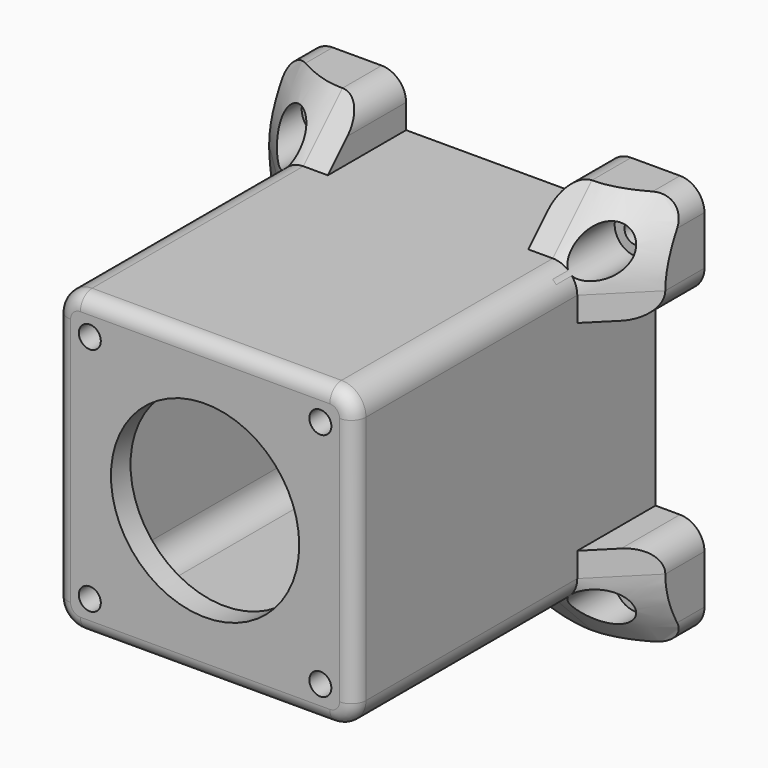
from build123d import *

# Parameters (mm, degrees)
F0_W          = 58
F0_H          = 58
F3_DEPTH      = 77
F4_DEPTH      = 5
F5_START      = 72
F0_R          = 19.25
F5_DEPTH      = 5
F6_DEPTH      = 91.6
F7_R          = 5
F8_D          = 4.5
F9_R          = 3
F10_T4_ANGLE  = 90
F10_T10_ANGLE = 90
F10_T16_ANGLE = 90
F10_T22_ANGLE = 90
F10_T28_DEPTH = 5
F10_T33_DEPTH = 5
F10_T38_DEPTH = 5
F10_T43_DEPTH = 5
F10_T48_DEPTH = 5
F10_T53_DEPTH = 5
F10_T58_DEPTH = 5
F10_T63_DEPTH = 5
F11_D         = 4.5
F13_START     = 7
F12_R         = 4.25
F13_DEPTH     = 17
F14_R         = 5


# Not quite as in the source:
# - a fillet or chamfer that OpenCascade refuses, or shapes differently, is made with other operations: its cross-section is extruded or revolved along the edge and cut away or added


with BuildPart() as f3:
    # F0 (on Front) → F3 (new body)
    with BuildSketch(Plane.XZ):
        Polygon((-30.5, -20.5), (-30.5, -30.5), (-20.5, -30.5), (20.5, -30.5), (30.5, -30.5), (30.5, -20.5), (30.5, 20.5), (30.5, 30.5), (20.5, 30.5), (-20.5, 30.5), (-30.5, 30.5), (-30.5, 20.5), align=None)
        Rectangle(F0_W, F0_H, mode=Mode.SUBTRACT)
    extrude(amount=F3_DEPTH)

    # F0 (on Front) → F4 (join)
    with BuildSketch(Plane.XZ):
        Polygon((-40.5, 20.5), (-30.5, 20.5), (-30.5, 30.5), (-20.5, 30.5), (-20.5, 40.5), (-40.5, 40.5), align=None)
        Polygon((30.5, 30.5), (30.5, 20.5), (40.5, 20.5), (40.5, 40.5), (20.5, 40.5), (20.5, 30.5), align=None)
        Polygon((30.5, -30.5), (20.5, -30.5), (20.5, -40.5), (40.5, -40.5), (40.5, -20.5), (30.5, -20.5), align=None)
        Polygon((-20.5, -30.5), (-30.5, -30.5), (-30.5, -20.5), (-40.5, -20.5), (-40.5, -40.5), (-20.5, -40.5), align=None)
    extrude(amount=F4_DEPTH)

    # F0 (on Front) → F5 (join)
    with BuildSketch(Plane.XZ.offset(F5_START)):
        Polygon((-30.5, -20.5), (-30.5, -30.5), (-20.5, -30.5), (20.5, -30.5), (30.5, -30.5), (30.5, -20.5), (30.5, 20.5), (30.5, 30.5), (20.5, 30.5), (-20.5, 30.5), (-30.5, 30.5), (-30.5, 20.5), align=None)
        Rectangle(F0_W, F0_H, mode=Mode.SUBTRACT)
        Rectangle(F0_W, F0_H)
        Circle(F0_R, mode=Mode.SUBTRACT)
    extrude(amount=F5_DEPTH)

    # F0 (on Front) → F6 (cut)
    with BuildSketch(Plane.XZ):
        Circle(F0_R)
    extrude(amount=F6_DEPTH, mode=Mode.SUBTRACT)

    # F7
    f7_edges = [f3.edges().sort_by_distance(p)[0] for p in [
        (-30.5, -41, 30.5),
        (-30.5, -41, -30.5),
        (30.5, -41, -30.5),
        (30.5, -41, 30.5),
        (-29, -36, -29),
        (-29, -36, 29),
        (29, -36, 29),
        (29, -36, -29),
    ]]
    fillet(f7_edges, radius=F7_R)

    # F8 (through all)
    with Locations(Plane(origin=(0, 0, 0), x_dir=(1, 0, 0), z_dir=(0, 1, 0))):
        with Locations((23.57, -23.57), (-23.57, 23.57), (-23.57, -23.57), (23.57, 23.57)):
            Hole(F8_D / 2)

    # F9
    f9_edges = [f3.edges().sort_by_distance(p)[0] for p in [
        (-30.5, -77, 0),
    ]]
    fillet(f9_edges, radius=F9_R)

    # F10: chamfer of 15 on 4 edges, made by hand


with BuildPart() as f10_tool2:
    # F10_s3 → F10_t4 (revolve)
    with BuildSketch(Plane.XY.offset(-25.5)):
        Polygon((30.5, -20), (45.5, -5), (30.5, -5), align=None)
    revolve(axis=Axis((25.5, -5, -25.5), (0, 1, 0)), revolution_arc=F10_T4_ANGLE)

    split(bisect_by=Plane.XY.offset(-40.5), keep=Keep.TOP)

    split(bisect_by=Plane.YZ.offset(40.5), keep=Keep.BOTTOM)


with BuildPart() as f3_1:
    add(f3.part)

    # F10_t1: union F10_tool2
    add(f10_tool2.part)


with BuildPart() as f10_tool8:
    # F10_s9 → F10_t10 (revolve)
    with BuildSketch(Plane.XY.offset(25.5)):
        Polygon((30.5, -20), (45.5, -5), (30.5, -5), align=None)
    revolve(axis=Axis((25.5, -5, 25.5), (0, -1, 0)), revolution_arc=F10_T10_ANGLE)

    split(bisect_by=Plane.YZ.offset(40.5), keep=Keep.BOTTOM)

    split(bisect_by=Plane.XY.offset(40.5), keep=Keep.BOTTOM)


with BuildPart() as f3_2:
    add(f3_1.part)

    # F10_t7: union F10_tool8
    add(f10_tool8.part)


with BuildPart() as f10_tool14:
    # F10_s15 → F10_t16 (revolve)
    with BuildSketch(Plane.XY.offset(25.5)):
        Polygon((-30.5, -20), (-45.5, -5), (-30.5, -5), align=None)
    revolve(axis=Axis((-25.5, -5, 25.5), (0, 1, 0)), revolution_arc=F10_T16_ANGLE)

    split(bisect_by=Plane.YZ.offset(-40.5), keep=Keep.TOP)

    split(bisect_by=Plane.XY.offset(40.5), keep=Keep.BOTTOM)


with BuildPart() as f3_3:
    add(f3_2.part)

    # F10_t13: union F10_tool14
    add(f10_tool14.part)


with BuildPart() as f10_tool20:
    # F10_s21 → F10_t22 (revolve)
    with BuildSketch(Plane.XY.offset(-25.5)):
        Polygon((-30.5, -20), (-45.5, -5), (-30.5, -5), align=None)
    revolve(axis=Axis((-25.5, -5, -25.5), (0, -1, 0)), revolution_arc=F10_T22_ANGLE)

    split(bisect_by=Plane.XY.offset(-40.5), keep=Keep.TOP)

    split(bisect_by=Plane.YZ.offset(-40.5), keep=Keep.TOP)


with BuildPart() as f3_4:
    add(f3_3.part)

    # F10_t19: union F10_tool20
    add(f10_tool20.part)


with BuildPart() as f10_tool26:
    # F10_s27 → F10_t28 (new body)
    with BuildSketch(Plane.XY.offset(-25.5)):
        Polygon((-30.5, -20), (-45.5, -5), (-30.5, -5), align=None)
    extrude(amount=F10_T28_DEPTH)

    split(bisect_by=Plane.YZ.offset(-40.5), keep=Keep.TOP)


with BuildPart() as f3_5:
    add(f3_4.part)

    # F10_t25: union F10_tool26
    add(f10_tool26.part)


with BuildPart() as f10_tool31:
    # F10_s32 → F10_t33 (new body)
    with BuildSketch(Plane.YZ.offset(-20.5)):
        Polygon((-5, -45.5), (-20, -30.5), (-5, -30.5), align=None)
    extrude(amount=-F10_T33_DEPTH)

    split(bisect_by=Plane.XY.offset(-40.5), keep=Keep.TOP)


with BuildPart() as f3_6:
    add(f3_5.part)

    # F10_t30: union F10_tool31
    add(f10_tool31.part)


with BuildPart() as f10_tool36:
    # F10_s37 → F10_t38 (new body)
    with BuildSketch(Plane.XY.offset(20.5)):
        Polygon((-30.5, -20), (-45.5, -5), (-30.5, -5), align=None)
    extrude(amount=F10_T38_DEPTH)

    split(bisect_by=Plane.YZ.offset(-40.5), keep=Keep.TOP)


with BuildPart() as f3_7:
    add(f3_6.part)

    # F10_t35: union F10_tool36
    add(f10_tool36.part)


with BuildPart() as f10_tool41:
    # F10_s42 → F10_t43 (new body)
    with BuildSketch(Plane.YZ.offset(-25.5)):
        Polygon((-5, 45.5), (-20, 30.5), (-5, 30.5), align=None)
    extrude(amount=F10_T43_DEPTH)

    split(bisect_by=Plane.XY.offset(40.5), keep=Keep.BOTTOM)


with BuildPart() as f3_8:
    add(f3_7.part)

    # F10_t40: union F10_tool41
    add(f10_tool41.part)


with BuildPart() as f10_tool46:
    # F10_s47 → F10_t48 (new body)
    with BuildSketch(Plane.XY.offset(25.5)):
        Polygon((30.5, -20), (45.5, -5), (30.5, -5), align=None)
    extrude(amount=-F10_T48_DEPTH)

    split(bisect_by=Plane.YZ.offset(40.5), keep=Keep.BOTTOM)


with BuildPart() as f3_9:
    add(f3_8.part)

    # F10_t45: union F10_tool46
    add(f10_tool46.part)


with BuildPart() as f10_tool51:
    # F10_s52 → F10_t53 (new body)
    with BuildSketch(Plane.YZ.offset(20.5)):
        Polygon((-20, 30.5), (-5, 45.5), (-5, 30.5), align=None)
    extrude(amount=F10_T53_DEPTH)

    split(bisect_by=Plane.XY.offset(40.5), keep=Keep.BOTTOM)


with BuildPart() as f3_10:
    add(f3_9.part)

    # F10_t50: union F10_tool51
    add(f10_tool51.part)


with BuildPart() as f10_tool56:
    # F10_s57 → F10_t58 (new body)
    with BuildSketch(Plane.XY.offset(-20.5)):
        Polygon((30.5, -20), (45.5, -5), (30.5, -5), align=None)
    extrude(amount=-F10_T58_DEPTH)

    split(bisect_by=Plane.YZ.offset(40.5), keep=Keep.BOTTOM)


with BuildPart() as f3_11:
    add(f3_10.part)

    # F10_t55: union F10_tool56
    add(f10_tool56.part)


with BuildPart() as f10_tool61:
    # F10_s62 → F10_t63 (new body)
    with BuildSketch(Plane.YZ.offset(25.5)):
        Polygon((-20, -30.5), (-5, -45.5), (-5, -30.5), align=None)
    extrude(amount=-F10_T63_DEPTH)

    split(bisect_by=Plane.XY.offset(-40.5), keep=Keep.TOP)


with BuildPart() as f3_12:
    add(f3_11.part)

    # F10_t60: union F10_tool61
    add(f10_tool61.part)

    # F11 (through all)
    with Locations(Plane(origin=(0, 0, 0), x_dir=(1, 0, 0), z_dir=(0, 1, 0))):
        with Locations((-32, 32), (32, 32), (32, -32), (-32, -32)):
            Hole(F11_D / 2)

    # F12 (on Front) → F13 (cut)
    with BuildSketch(Plane.XZ.offset(F13_START)):
        with Locations((-32, 32)):
            Circle(F12_R)
        with Locations((32, -32)):
            Circle(F12_R)
        with Locations((32, 32)):
            Circle(F12_R)
        with Locations((-32, -32)):
            Circle(F12_R)
    extrude(amount=F13_DEPTH, mode=Mode.SUBTRACT)

    # F14
    f14_edges = [f3_12.edges().sort_by_distance(p)[0] for p in [
        (40.5, -2.5, 40.5),
        (20.5, -5, 40.5),
        (40.5, -5, 20.5),
        (40.5, -5, -20.5),
        (40.5, -2.5, -40.5),
        (20.5, -5, -40.5),
        (-20.5, -5, -40.5),
        (-40.5, -2.5, -40.5),
        (-40.5, -5, -20.5),
        (-40.5, -5, 20.5),
        (-40.5, -2.5, 40.5),
        (-20.5, -5, 40.5),
    ]]
    fillet(f14_edges, radius=F14_R)


solid = f3_12.part
